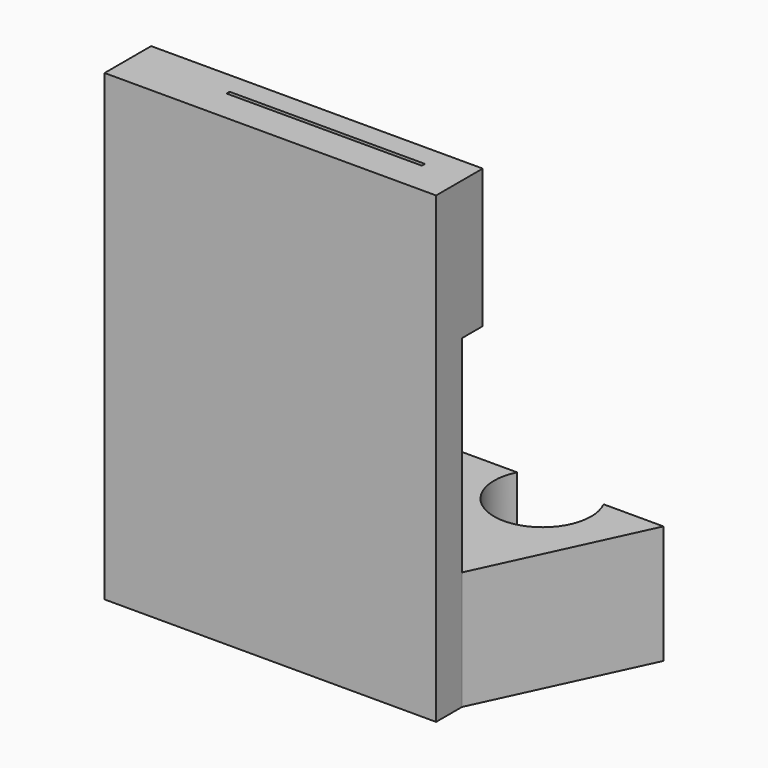
from build123d import *

# Parameters (mm, degrees)
F0_R           = 7.5
F1_DEPTH       = 7.6
F1_DEPTH_BACK  = 17.3
F2_DEPTH       = 6.8
F4_DEPTH       = 4.4
F4_DEPTH_BACK  = 13.9
F6_W           = 51.2241850299
F6_H           = 71.6110350132
F7_DEPTH       = 5
F10_DEPTH      = 0.6
F11_W          = 51.2241850299
F11_H          = 21.4426852763
F12_DEPTH      = 4
F15_R          = 5
F16_DEPTH      = 25
F16_DEPTH_BACK = 25


with BuildPart() as f1:
    # F0 (on Top) → F1 (new body, two sides)
    with BuildSketch(Plane.XY) as f1_sk:
        with Locations((-21.15, 0)):
            Circle(F0_R)
    extrude(amount=F1_DEPTH)
    extrude(f1_sk.sketch, amount=-F1_DEPTH_BACK)


with BuildPart() as f1b:
    # F0 (on Top) → F1, piece 2 (new body, two sides)
    with BuildSketch(Plane.XY) as f1_2_sk:
        with Locations((21.15, 0)):
            Circle(F0_R)
    extrude(amount=F1_DEPTH)
    extrude(f1_2_sk.sketch, amount=-F1_DEPTH_BACK)


with BuildPart() as f2:
    # F0 (on Top) → F2 (new body)
    with BuildSketch(Plane.XY):
        Polygon((-6.5, 4.1165491707), (-6.5, 0), (-6.5, -4.1165491707), (0, -7.19), (6.5, -4.1165491707), (6.5, 0), (6.5, 4.1165491707), (0, 7.19), align=None)
    extrude(amount=-F2_DEPTH)


with BuildPart() as f4:
    # F3 (on Top) → F4 (new body, two sides)
    with BuildSketch(Plane.XY) as f4_sk:
        Polygon((-25.612092515, -21.15), (25.612092515, -21.15), (37.0736953387, 3.4294865757), (-37.0736953387, 3.4294865757), align=None)
    extrude(amount=F4_DEPTH)
    extrude(f4_sk.sketch, amount=-F4_DEPTH_BACK)

    # F5: cut F1, F2, F1b
    add(f1.part, mode=Mode.SUBTRACT)
    add(f2.part, mode=Mode.SUBTRACT)
    add(f1b.part, mode=Mode.SUBTRACT)

    # F6 (on face) → F7 (join)
    with BuildSketch(Plane.XZ.offset(21.15)):
        with Locations((0, 21.9055175066)):
            Rectangle(F6_W, F6_H)
    extrude(amount=F7_DEPTH)

    # F11 (on face) → F12 (join)
    with BuildSketch(Plane(origin=(0, -21.15, 0), x_dir=(-1, 0, 0), z_dir=(0, 1, 0))):
        with Locations((0, 46.9896923751)):
            Rectangle(F11_W, F11_H)
    extrude(amount=F12_DEPTH)


with BuildPart() as f10:
    # F9 (on offset) → F10 (new body)
    with BuildSketch(Plane(origin=(0, -20.55, 0), x_dir=(-1, 0, 0), z_dir=(0, 1, 0))):
        Polygon((-20, 58.7664473951), (-10.2, 40.7664473951), (20, 40.7664473951), (10.2, 58.7664473951), align=None)
    extrude(amount=-F10_DEPTH)


with BuildPart() as f4_1:
    add(f4.part)

    # F13: cut F10
    add(f10.part, mode=Mode.SUBTRACT)

    # F15 (on face) → F16 (cut, two sides)
    with BuildSketch(Plane(origin=(0, 0, -13.9), x_dir=(1, 0, 0), z_dir=(0, 0, -1))) as f16_sk:
        Circle(F15_R)
    extrude(amount=-F16_DEPTH, mode=Mode.SUBTRACT)
    extrude(f16_sk.sketch, amount=F16_DEPTH_BACK, mode=Mode.SUBTRACT)


solid = f4_1.part
